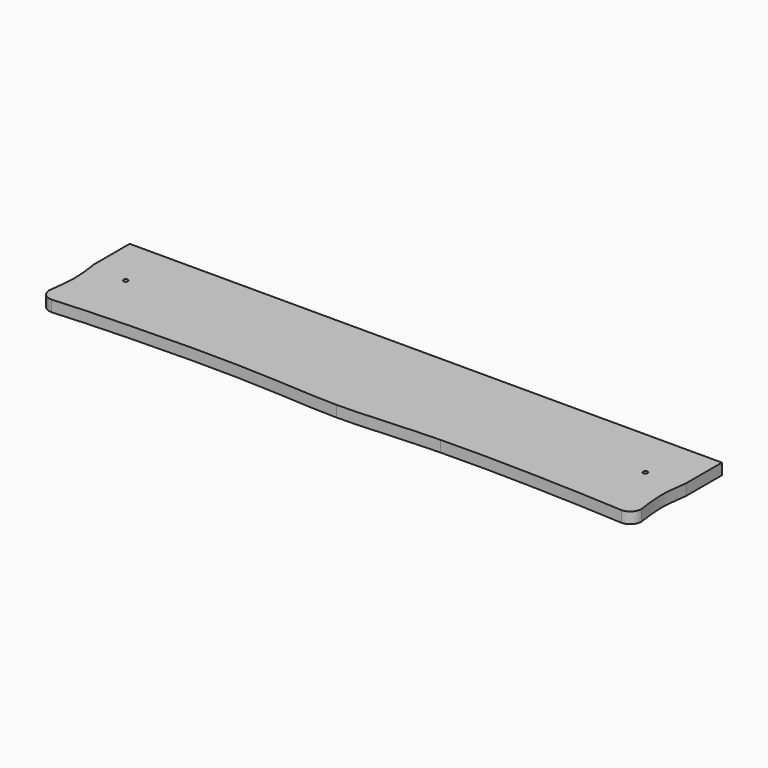
from build123d import *

# Parameters (mm, degrees)
F0_W     = 673.1
F0_H     = 127
F1_DEPTH = 12.7
F3_DEPTH = 12.7
F4_R     = 12.69999
F6_DEPTH = 12.7


# Not quite as in the source:
# - a fillet or chamfer is up to 0.001 mm smaller than in the source, because OpenCascade refuses the exact size
# - ends of sketch curves that miss each other by under 0.0002 mm in the source are joined


with BuildPart() as f1:
    # F0 (on Top) → F1 (new body)
    with BuildSketch(Plane.XY):
        with Locations((-336.55, 63.5)):
            Rectangle(F0_W, F0_H)
    extrude(amount=F1_DEPTH)

    # F2 (on face) → F3 (cut)
    with BuildSketch(Plane.XY.offset(12.7)):
        with BuildLine():
            Line((-660.4, 0), (-450.85, 0))
            Line((-450.85, 0), (-450.85, 5.08))
            add(Edge.make_bspline(
                [(-660.4, 0), (-618.4280983715, 3.4161410723), (-518.2102721788, 6.7061283939), (-450.85, 5.08)],
                knots=[0, 0, 0, 0, 0.2875538304, 0.2875538304, 0.2875538304, 0.2875538304], degree=3))
        make_face()
        with BuildLine():
            Line((-450.85, 5.08), (-450.85, 0))
            Line((-450.85, 0), (-336.6277222604, 0))
            add(Edge.make_bspline(
                [(-450.85, 5.08), (-401.1233292925, 3.8795602073), (-369.3029781403, -5.9421e-06), (-336.6277222604, 0)],
                knots=[0.2875538304, 0.2875538304, 0.2875538304, 0.2875538304, 0.4998316935, 0.4998316935, 0.4998316935, 0.4998316935], degree=3))
        make_face()
        with BuildLine():
            add(Edge.make_bspline(
                [(-336.6277222604, -7.3164e-06), (-336.6018153808, -7.3175e-06), (-303.8740668477, 0.0030721325), (-270.2737779375, 3.9032465323), (-222.25, 5.08)],
                knots=[0.4998316935, 0.4998316935, 0.4998316935, 0.4998316935, 0.5, 0.7124461696, 0.7124461696, 0.7124461696, 0.7124461696], degree=3))
            Line((-336.6277222604, -7.3164e-06), (-222.25, 0))
            Line((-222.25, 0), (-222.25, 5.08))
        make_face()
        with BuildLine():
            add(Edge.make_bspline(
                [(-222.25, 5.08), (-157.2480217343, 6.6727797981), (-65.7725673543, 3.2817360247), (-12.7, 0)],
                knots=[0.7124461696, 0.7124461696, 0.7124461696, 0.7124461696, 1, 1, 1, 1], degree=3))
            Line((-222.25, 5.08), (-222.25, 0))
            Line((-222.25, 0), (-12.7, 0))
        make_face()
        with BuildLine():
            add(Edge.make_bspline(
                [(0, 76.2), (-1.5243553143, 65.6073133136), (-3.0487106286, 55.0146266272), (-3.048, 44.4275960326)],
                knots=[0, 0, 0, 0, 0.5001747983, 0.5001747983, 0.5001747983, 0.5001747983], degree=3))
            Line((-3.048, 44.4275960326), (0, 44.4275960326))
            Line((0, 44.4275960326), (0, 76.2))
        make_face()
        with BuildLine():
            add(Edge.make_bspline(
                [(-3.048, 44.4275960326), (-3.0472898681, 33.8479652297), (-1.523644934, 23.2739826149), (0, 12.7)],
                knots=[0.5001747983, 0.5001747983, 0.5001747983, 0.5001747983, 1, 1, 1, 1], degree=3))
            Line((0, 12.7), (0, 44.4275960326))
            Line((0, 44.4275960326), (-3.048, 44.4275960326))
        make_face()
        with BuildLine():
            Line((-673.1, 45.72), (-670.052, 45.72))
            add(Edge.make_bspline(
                [(-673.1, 76.2), (-671.5957505111, 66.1426093711), (-670.0915010221, 56.0852187422), (-670.052, 45.72)],
                knots=[0, 0, 0, 0, 0.4900875678, 0.4900875678, 0.4900875678, 0.4900875678], degree=3))
            Line((-673.1, 76.2), (-673.1, 45.72))
        make_face()
        with BuildLine():
            Line((-673.1, 45.72), (-673.1, 12.7))
            add(Edge.make_bspline(
                [(-670.052, 45.72), (-670.0109010952, 34.9354907678), (-671.5554505476, 23.8177453839), (-673.1, 12.7)],
                knots=[0.4900875678, 0.4900875678, 0.4900875678, 0.4900875678, 1, 1, 1, 1], degree=3))
            Line((-670.052, 45.72), (-673.1, 45.72))
        make_face()
    extrude(amount=-F3_DEPTH, mode=Mode.SUBTRACT)

    # F4 (radius 12.7 in the source; OpenCascade refuses exactly that, so slightly less here)
    f4_edges = [f1.edges().sort_by_distance(p)[0] for p in [
        (-673.1, 0, 6.35),
        (0, 0, 6.35),
    ]]
    fillet(f4_edges, radius=F4_R)

    # F5 (on face) → F6 (cut)
    with BuildSketch(Plane(origin=(0, 0, 0), x_dir=(1, 0, 0), z_dir=(0, 0, -1))):
        with BuildLine():
            ThreePointArc((-38.69436, -69.85), (-43.0997880438, -68.0252119562), (-41.275, -72.43064))
            ThreePointArc((-41.275, -72.43064), (-39.4502119562, -71.6747880438), (-38.69436, -69.85))
        make_face()
        with BuildLine():
            ThreePointArc((-629.24436, -69.85), (-633.6497880438, -68.0252119562), (-631.825, -72.43064))
            ThreePointArc((-631.825, -72.43064), (-630.0002119562, -71.6747880438), (-629.24436, -69.85))
        make_face()
    extrude(amount=-F6_DEPTH, mode=Mode.SUBTRACT)


solid = f1.part
